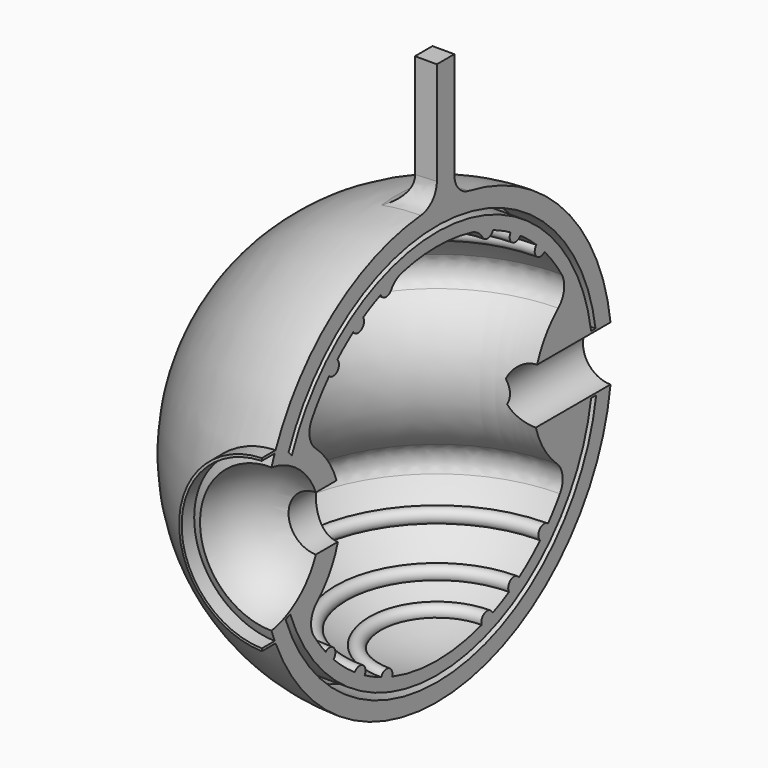
from build123d import *

# Parameters (mm, degrees)
F8_W      = 23.3316195624
F8_H      = 6.25
F10_R     = 5
F11_R     = 6.25
F12_DEPTH = 33.3333333333
F14_DEPTH = 10
F15_DEPTH = 10
F17_W     = 5
F17_H     = 5
F18_DEPTH = 3.3333333333
F19_W     = 5
F19_H     = 5
F20_DEPTH = 25
F22_DEPTH = 5
F23_R     = 5


with BuildPart() as f2:
    # F1 (on Top) → F2 (revolve)
    with BuildSketch(Plane.XY):
        with BuildLine():
            Line((0, 0), (0, 50))
            ThreePointArc((0, 50), (-35.2493093402, 35.2493093402), (-50, 0))
            Line((-50, 0), (0, 0))
        make_face()
    revolve(axis=Axis((-25, 0, 0), (1, 0, 0)))

    # F4 (on offset) → F5 (revolve, cut)
    with BuildSketch(Plane.XZ.offset(50)):
        with BuildLine():
            Line((0, -16.6666666667), (0, 16.6666666667))
            ThreePointArc((0, 16.6666666667), (-16.6666666667, 0), (0, -16.6666666667))
        make_face()
    revolve(axis=Axis((0, -50, -1.9737724215), (0, 0, -1)), mode=Mode.SUBTRACT)

    # F6 (on face) → F7 (revolve, cut)
    with BuildSketch(Plane.YZ):
        with BuildLine():
            ThreePointArc((-37.8466364555, 17.4282305503), (-27.4757859957, -0.3256138007), (-37.422983522, -18.3202460524))
            ThreePointArc((-37.422983522, -18.3202460524), (-34.8598457139, -22.8232834605), (-31.7576392855, -26.9733842541))
            ThreePointArc((-31.7576392855, -26.9733842541), (-29.4273730681, -27.0929827504), (-29.5003423179, -29.4251748379))
            ThreePointArc((-29.5003423179, -29.4251748379), (-26.5938204324, -32.0761566576), (-23.4502430753, -34.4412138407))
            ThreePointArc((-23.4502430753, -34.4412138407), (-21.1719454891, -33.937423653), (-20.6226901178, -36.2051897304))
            ThreePointArc((-20.6226901178, -36.2051897304), (-18.3031433498, -37.4313512263), (-15.9110236835, -38.5090955029))
            ThreePointArc((-15.9110236835, -38.5090955029), (-13.7839095821, -37.550017798), (-12.7824814299, -39.65752488))
            ThreePointArc((-12.7824814299, -39.65752488), (-6.4697079189, -41.1613166766), (0, -41.6666666667))
            Line((0, -41.6666666667), (0, 41.6666666667))
            ThreePointArc((0, 41.6666666667), (-6.533606679, 41.1512222768), (-12.9055632344, 39.6176418873))
            ThreePointArc((-12.9055632344, 39.6176418873), (-13.900442387, 37.5070353593), (-16.0305243346, 38.4595033856))
            ThreePointArc((-16.0305243346, 38.4595033856), (-18.5825324003, 37.2934391107), (-21.0502773816, 35.9582665498))
            ThreePointArc((-21.0502773816, 35.9582665498), (-21.5726209218, 33.6841509699), (-23.8567285038, 34.1609077193))
            ThreePointArc((-23.8567285038, 34.1609077193), (-26.2072797797, 32.3927398912), (-28.4272331294, 30.4631503249))
            ThreePointArc((-28.4272331294, 30.4631503249), (-28.4378626812, 28.1298412033), (-30.7709176854, 28.0938024466))
            ThreePointArc((-30.7709176854, 28.0938024466), (-34.7207544566, 23.0343291865), (-37.8466364555, 17.4282305503))
        make_face()
    revolve(axis=Axis((0, 0, 1.4037434012), (0, 0, -1)), mode=Mode.SUBTRACT)

    # F8 (on face) → F9 (revolve, cut)
    with BuildSketch(Plane.YZ):
        with Locations((38.6982297662, 3.125)):
            Rectangle(F8_W, F8_H)
    revolve(axis=Axis((0, 36.5484141222, 0), (0, -1, 0)), mode=Mode.SUBTRACT)

    # F10
    f10_edges = [f2.edges().sort_by_distance(p)[0] for p in [
        (-37.422984, 0, -18.320246),
        (-37.846636, 0, 17.428231),
        (-12.905563, 0, 39.617642),
    ]]
    fillet(f10_edges, radius=F10_R)

    # F11 (on offset) → F12 (cut)
    with BuildSketch(Plane.XZ.offset(50)):
        Circle(F11_R)
    extrude(amount=-F12_DEPTH, mode=Mode.SUBTRACT)

    # F13 (on face) → F14 (cut)
    with BuildSketch(Plane.YZ):
        with BuildLine():
            ThreePointArc((-41.4440813955, 16.4335549531), (5.0165595874, 44.3002002368), (44.0693897293, 6.75))
            Line((44.0693897293, 6.75), (45.3335631122, 6.75))
            ThreePointArc((45.3335631122, 6.75), (5.5806134402, 45.4923202099), (-42.3578890966, 17.5072463776))
            Line((-42.3578890966, 17.5072463776), (-41.4440813955, 16.4335549531))
        make_face()
    extrude(amount=-F14_DEPTH, mode=Mode.SUBTRACT)

    # F13 (on face) → F15 (cut)
    with BuildSketch(Plane.YZ):
        with BuildLine():
            ThreePointArc((-43.213327735, -15.8020152475), (4.6699173407, -45.7743077703), (45.5140953971, -6.75))
            Line((45.5140953971, -6.75), (44.0693897293, -6.75))
            ThreePointArc((44.0693897293, -6.75), (4.4230742659, -44.3633860875), (-41.8691718428, -15.318161127))
            Line((-41.8691718428, -15.318161127), (-43.213327735, -15.8020152475))
        make_face()
    extrude(amount=-F15_DEPTH, mode=Mode.SUBTRACT)

    # F17 (on offset) → F18 (join, symmetric)
    with BuildSketch(Plane.XY.offset(50)):
        with Locations((-2.5, 2.5)):
            Rectangle(F17_W, F17_H)
    extrude(amount=F18_DEPTH, both=True)

    # F19 (on face) → F20 (join)
    with BuildSketch(Plane.XY.offset(53.3333333333)):
        with Locations((-2.5, 2.5)):
            Rectangle(F19_W, F19_H)
    extrude(amount=F20_DEPTH)

    # F21 (on offset) → F22 (join)
    with BuildSketch(Plane.XZ.offset(50)):
        with BuildLine():
            ThreePointArc((0, -18.8601790593), (-18.327349043, 0), (0, 18.8601790593))
            Line((0, 18.8601790593), (0, 19.4318354018))
            ThreePointArc((0, 19.4318354018), (-18.8987776144, 0), (0, -19.4318354018))
            Line((0, -19.4318354018), (0, -18.8601790593))
        make_face()
    extrude(amount=-F22_DEPTH)

    # F23
    f23_edges = [f2.edges().sort_by_distance(p)[0] for p in [
        (-2.503584, 5, 49.668523),
        (-5, 2.503175, 49.651691),
        (-2.503548, 0, 49.919559),
    ]]
    fillet(f23_edges, radius=F23_R)


solid = f2.part
